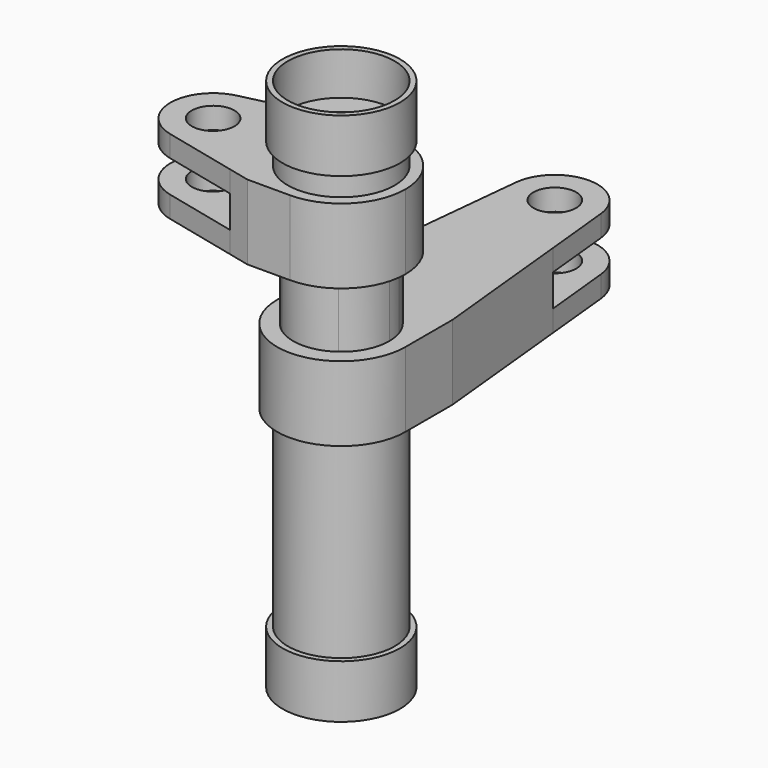
from build123d import *

# Parameters (mm, degrees)
F1_START       = 20
F0_R           = 5.5
F0_R_2         = 5
F1_DEPTH       = 5
F2_START       = 18
F0_R_3         = 2.75
F2_DEPTH       = 3
F3_START       = 14.5
F3_DEPTH       = 3.5
F4_START       = 11
F0_R_4         = 2
F4_DEPTH       = 7
F5_START       = 13
F5_DEPTH       = 3
F6_START       = 11
F6_DEPTH       = 3.5
F7_START       = 5
F7_DEPTH       = 6
F8_START       = 1.5
F8_DEPTH       = 3.5
F9_DEPTH       = 5
F9_DEPTH_BACK  = 2
F10_DEPTH      = 3
F11_DEPTH      = 1.5
F11_DEPTH_BACK = 2
F12_START      = -2
F12_DEPTH      = 19
F13_START      = -20
F13_DEPTH      = 5


# Not quite as in the source:
# - a feature names something its author has since deleted; it is built from what else it names


with BuildPart() as f1:
    # F0 (on Top) → F1 (new body)
    with BuildSketch(Plane.XY.offset(F1_START)):
        Circle(F0_R)
        Circle(F0_R_2, mode=Mode.SUBTRACT)
    extrude(amount=F1_DEPTH)

    # F0 (on Top) → F2 (join)
    with BuildSketch(Plane.XY.offset(F2_START)):
        Circle(F0_R_2)
        with BuildLine():
            ThreePointArc((4.2797543233, 1.3905764747), (4.4445975327, 0.7039550927), (4.5, 0))
            ThreePointArc((4.5, 0), (4.0095293588, -2.0429572488), (2.6450336353, -3.6405764747))
            ThreePointArc((2.6450336353, -3.6405764747), (0, -4.5), (-2.6450336353, -3.6405764747))
            ThreePointArc((-2.6450336353, -3.6405764747), (-4.2797543233, -1.3905764747), (-4.2797543233, 1.3905764747))
            ThreePointArc((-4.2797543233, 1.3905764747), (-2.6450336353, 3.6405764747), (0, 4.5))
            ThreePointArc((0, 4.5), (2.6450336353, 3.6405764747), (4.2797543233, 1.3905764747))
        make_face(mode=Mode.SUBTRACT)
        Polygon((2.6450336353, -3.6405764747), (4.2797543233, 1.3905764747), (0, 4.5), (-4.2797543233, 1.3905764747), (-2.6450336353, -3.6405764747), align=None)
        Circle(F0_R_3, mode=Mode.SUBTRACT)
        with BuildLine():
            Line((-4.2797543233, 1.3905764747), (0, 4.5))
            ThreePointArc((0, 4.5), (-2.6450336353, 3.6405764747), (-4.2797543233, 1.3905764747))
        make_face()
        with BuildLine():
            Line((0, 4.5), (4.2797543233, 1.3905764747))
            ThreePointArc((4.2797543233, 1.3905764747), (2.6450336353, 3.6405764747), (0, 4.5))
        make_face()
        with BuildLine():
            ThreePointArc((2.6450336353, -3.6405764747), (4.0095293588, -2.0429572488), (4.5, 0))
            ThreePointArc((4.5, 0), (4.4445975327, 0.7039550927), (4.2797543233, 1.3905764747))
            Line((4.2797543233, 1.3905764747), (2.6450336353, -3.6405764747))
        make_face()
        with BuildLine():
            ThreePointArc((-4.2797543233, 1.3905764747), (-4.2797543233, -1.3905764747), (-2.6450336353, -3.6405764747))
            Line((-2.6450336353, -3.6405764747), (-4.2797543233, 1.3905764747))
        make_face()
        with BuildLine():
            ThreePointArc((-2.6450336353, -3.6405764747), (0, -4.5), (2.6450336353, -3.6405764747))
            Line((2.6450336353, -3.6405764747), (-2.6450336353, -3.6405764747))
        make_face()
    extrude(amount=F2_DEPTH)

    # F0 (on Top) → F3 (join)
    with BuildSketch(Plane.XY.offset(F3_START)):
        Polygon((2.6450336353, -3.6405764747), (4.2797543233, 1.3905764747), (0, 4.5), (-4.2797543233, 1.3905764747), (-2.6450336353, -3.6405764747), align=None)
        Circle(F0_R_3, mode=Mode.SUBTRACT)
    extrude(amount=F3_DEPTH)


with BuildPart() as f4:
    # F0 (on Top) → F4 (new body)
    with BuildSketch(Plane.XY.offset(F4_START)):
        with BuildLine():
            ThreePointArc((6, 0), (4.2426406871, 4.2426406871), (0, 6))
            ThreePointArc((0, 6), (-4.2426406871, 4.2426406871), (-6, 0))
            ThreePointArc((-6, 0), (-4.2426406871, -4.2426406871), (0, -6))
            ThreePointArc((0, -6), (4.2426406871, -4.2426406871), (6, 0))
        make_face()
        Circle(F0_R, mode=Mode.SUBTRACT)
        Circle(F0_R)
        Circle(F0_R_2, mode=Mode.SUBTRACT)
        with BuildLine():
            Line((-6, -5.5275252317), (-6, 0))
            Line((-6, 0), (-6, 5.5275252317))
            Line((-6, 5.5275252317), (-12.9196363336, 3.8928484448))
            ThreePointArc((-12.9196363336, 3.8928484448), (-16, 0), (-12.9196363336, -3.8928484448))
            Line((-12.9196363336, -3.8928484448), (-6, -5.5275252317))
        make_face()
        with Locations((-12, 0)):
            Circle(F0_R_4, mode=Mode.SUBTRACT)
        Circle(F0_R_2)
        with BuildLine():
            ThreePointArc((4.2797543233, 1.3905764747), (4.4445975327, 0.7039550927), (4.5, 0))
            ThreePointArc((4.5, 0), (4.0095293588, -2.0429572488), (2.6450336353, -3.6405764747))
            ThreePointArc((2.6450336353, -3.6405764747), (0, -4.5), (-2.6450336353, -3.6405764747))
            ThreePointArc((-2.6450336353, -3.6405764747), (-4.2797543233, -1.3905764747), (-4.2797543233, 1.3905764747))
            ThreePointArc((-4.2797543233, 1.3905764747), (-2.6450336353, 3.6405764747), (0, 4.5))
            ThreePointArc((0, 4.5), (2.6450336353, 3.6405764747), (4.2797543233, 1.3905764747))
        make_face(mode=Mode.SUBTRACT)
        with BuildLine():
            ThreePointArc((-6, 0), (-4.2426406871, 4.2426406871), (0, 6))
            Line((0, 6), (-4, 6))
            Line((-4, 6), (-6, 5.5275252317))
            Line((-6, 5.5275252317), (-6, 0))
        make_face()
        with BuildLine():
            ThreePointArc((0, -6), (-4.2426406871, -4.2426406871), (-6, 0))
            Line((-6, 0), (-6, -5.5275252317))
            Line((-6, -5.5275252317), (-4, -6))
            Line((-4, -6), (0, -6))
        make_face()
        with BuildLine():
            ThreePointArc((-4.2797543233, 1.3905764747), (-4.2797543233, -1.3905764747), (-2.6450336353, -3.6405764747))
            Line((-2.6450336353, -3.6405764747), (-4.2797543233, 1.3905764747))
        make_face()
        with BuildLine():
            ThreePointArc((2.6450336353, -3.6405764747), (4.0095293588, -2.0429572488), (4.5, 0))
            ThreePointArc((4.5, 0), (4.4445975327, 0.7039550927), (4.2797543233, 1.3905764747))
            Line((4.2797543233, 1.3905764747), (2.6450336353, -3.6405764747))
        make_face()
        with BuildLine():
            ThreePointArc((-2.6450336353, -3.6405764747), (0, -4.5), (2.6450336353, -3.6405764747))
            Line((2.6450336353, -3.6405764747), (-2.6450336353, -3.6405764747))
        make_face()
        with BuildLine():
            Line((0, 4.5), (4.2797543233, 1.3905764747))
            ThreePointArc((4.2797543233, 1.3905764747), (2.6450336353, 3.6405764747), (0, 4.5))
        make_face()
        with BuildLine():
            Line((-4.2797543233, 1.3905764747), (0, 4.5))
            ThreePointArc((0, 4.5), (-2.6450336353, 3.6405764747), (-4.2797543233, 1.3905764747))
        make_face()
    extrude(amount=F4_DEPTH)

    # F0 (on Top) → F5 (cut)
    with BuildSketch(Plane.XY.offset(F5_START)):
        with BuildLine():
            Line((-6, -5.5275252317), (-6, 0))
            Line((-6, 0), (-6, 5.5275252317))
            Line((-6, 5.5275252317), (-12.9196363336, 3.8928484448))
            ThreePointArc((-12.9196363336, 3.8928484448), (-16, 0), (-12.9196363336, -3.8928484448))
            Line((-12.9196363336, -3.8928484448), (-6, -5.5275252317))
        make_face()
        with Locations((-12, 0)):
            Circle(F0_R_4, mode=Mode.SUBTRACT)
    extrude(amount=F5_DEPTH, mode=Mode.SUBTRACT)


with BuildPart() as f6:
    # F0 (on Top) → F6 (new body)
    with BuildSketch(Plane.XY.offset(F6_START)):
        Polygon((2.6450336353, -3.6405764747), (4.2797543233, 1.3905764747), (0, 4.5), (-4.2797543233, 1.3905764747), (-2.6450336353, -3.6405764747), align=None)
        Circle(F0_R_3, mode=Mode.SUBTRACT)
    extrude(amount=F6_DEPTH)

    # F0 (on Top) → F7 (join)
    with BuildSketch(Plane.XY.offset(F7_START)):
        with BuildLine():
            Line((0, 4.5), (4.2797543233, 1.3905764747))
            ThreePointArc((4.2797543233, 1.3905764747), (2.6450336353, 3.6405764747), (0, 4.5))
        make_face()
        Polygon((2.6450336353, -3.6405764747), (4.2797543233, 1.3905764747), (0, 4.5), (-4.2797543233, 1.3905764747), (-2.6450336353, -3.6405764747), align=None)
        Circle(F0_R_3, mode=Mode.SUBTRACT)
        with BuildLine():
            ThreePointArc((2.6450336353, -3.6405764747), (4.0095293588, -2.0429572488), (4.5, 0))
            ThreePointArc((4.5, 0), (4.4445975327, 0.7039550927), (4.2797543233, 1.3905764747))
            Line((4.2797543233, 1.3905764747), (2.6450336353, -3.6405764747))
        make_face()
        with BuildLine():
            Line((-4.2797543233, 1.3905764747), (0, 4.5))
            ThreePointArc((0, 4.5), (-2.6450336353, 3.6405764747), (-4.2797543233, 1.3905764747))
        make_face()
        with BuildLine():
            ThreePointArc((-2.6450336353, -3.6405764747), (0, -4.5), (2.6450336353, -3.6405764747))
            Line((2.6450336353, -3.6405764747), (-2.6450336353, -3.6405764747))
        make_face()
        with BuildLine():
            ThreePointArc((-4.2797543233, 1.3905764747), (-4.2797543233, -1.3905764747), (-2.6450336353, -3.6405764747))
            Line((-2.6450336353, -3.6405764747), (-4.2797543233, 1.3905764747))
        make_face()
    extrude(amount=F7_DEPTH)

    # F0 (on Top) → F8 (join)
    with BuildSketch(Plane.XY.offset(F8_START)):
        Polygon((2.6450336353, -3.6405764747), (4.2797543233, 1.3905764747), (0, 4.5), (-4.2797543233, 1.3905764747), (-2.6450336353, -3.6405764747), align=None)
        Circle(F0_R_3, mode=Mode.SUBTRACT)
    extrude(amount=F8_DEPTH)


with BuildPart() as f9:
    # F0 (on Top) → F9 (new body, two sides)
    with BuildSketch(Plane.XY) as f9_sk:
        with BuildLine():
            Line((-4, 6), (0, 6))
            ThreePointArc((0, 6), (4.2426406871, 4.2426406871), (6, 0))
            Line((6, 0), (6, 5.5275252317))
            Line((6, 5.5275252317), (4.6305157529, 19))
            Line((4.6305157529, 19), (-4.6305157529, 19))
            Line((-4.6305157529, 19), (-6, 5.5275252317))
            Line((-6, 5.5275252317), (-4, 6))
        make_face()
        with BuildLine():
            ThreePointArc((6, 0), (4.2426406871, 4.2426406871), (0, 6))
            ThreePointArc((0, 6), (-4.2426406871, 4.2426406871), (-6, 0))
            ThreePointArc((-6, 0), (-4.2426406871, -4.2426406871), (0, -6))
            ThreePointArc((0, -6), (4.2426406871, -4.2426406871), (6, 0))
        make_face()
        Circle(F0_R, mode=Mode.SUBTRACT)
        Circle(F0_R)
        Circle(F0_R_2, mode=Mode.SUBTRACT)
        Circle(F0_R_2)
        with BuildLine():
            ThreePointArc((4.2797543233, 1.3905764747), (4.4445975327, 0.7039550927), (4.5, 0))
            ThreePointArc((4.5, 0), (4.0095293588, -2.0429572488), (2.6450336353, -3.6405764747))
            ThreePointArc((2.6450336353, -3.6405764747), (0, -4.5), (-2.6450336353, -3.6405764747))
            ThreePointArc((-2.6450336353, -3.6405764747), (-4.2797543233, -1.3905764747), (-4.2797543233, 1.3905764747))
            ThreePointArc((-4.2797543233, 1.3905764747), (-2.6450336353, 3.6405764747), (0, 4.5))
            ThreePointArc((0, 4.5), (2.6450336353, 3.6405764747), (4.2797543233, 1.3905764747))
        make_face(mode=Mode.SUBTRACT)
        with BuildLine():
            Line((-3.9794931225, 25.4045175988), (-4.6305157529, 19))
            Line((-4.6305157529, 19), (4.6305157529, 19))
            Line((4.6305157529, 19), (3.9794931225, 25.4045175988))
            ThreePointArc((3.9794931225, 25.4045175988), (0, 29), (-3.9794931225, 25.4045175988))
        make_face()
        with Locations((0, 25)):
            Circle(F0_R_4, mode=Mode.SUBTRACT)
        with BuildLine():
            ThreePointArc((-6, 0), (-4.2426406871, 4.2426406871), (0, 6))
            Line((0, 6), (-4, 6))
            Line((-4, 6), (-6, 5.5275252317))
            Line((-6, 5.5275252317), (-6, 0))
        make_face()
        with BuildLine():
            ThreePointArc((2.6450336353, -3.6405764747), (4.0095293588, -2.0429572488), (4.5, 0))
            ThreePointArc((4.5, 0), (4.4445975327, 0.7039550927), (4.2797543233, 1.3905764747))
            Line((4.2797543233, 1.3905764747), (2.6450336353, -3.6405764747))
        make_face()
        with BuildLine():
            ThreePointArc((-4.2797543233, 1.3905764747), (-4.2797543233, -1.3905764747), (-2.6450336353, -3.6405764747))
            Line((-2.6450336353, -3.6405764747), (-4.2797543233, 1.3905764747))
        make_face()
        with BuildLine():
            Line((-4.2797543233, 1.3905764747), (0, 4.5))
            ThreePointArc((0, 4.5), (-2.6450336353, 3.6405764747), (-4.2797543233, 1.3905764747))
        make_face()
        with BuildLine():
            ThreePointArc((-2.6450336353, -3.6405764747), (0, -4.5), (2.6450336353, -3.6405764747))
            Line((2.6450336353, -3.6405764747), (-2.6450336353, -3.6405764747))
        make_face()
        with BuildLine():
            Line((0, 4.5), (4.2797543233, 1.3905764747))
            ThreePointArc((4.2797543233, 1.3905764747), (2.6450336353, 3.6405764747), (0, 4.5))
        make_face()
    extrude(amount=F9_DEPTH)
    extrude(f9_sk.sketch, amount=-F9_DEPTH_BACK)

    # F0 (on Top) → F10 (cut)
    with BuildSketch(Plane.XY):
        with BuildLine():
            Line((-3.9794931225, 25.4045175988), (-4.6305157529, 19))
            Line((-4.6305157529, 19), (4.6305157529, 19))
            Line((4.6305157529, 19), (3.9794931225, 25.4045175988))
            ThreePointArc((3.9794931225, 25.4045175988), (0, 29), (-3.9794931225, 25.4045175988))
        make_face()
        with Locations((0, 25)):
            Circle(F0_R_4, mode=Mode.SUBTRACT)
    extrude(amount=F10_DEPTH, mode=Mode.SUBTRACT)


with BuildPart() as f11:
    # F0 (on Top) → F11 (new body, two sides)
    with BuildSketch(Plane.XY) as f11_sk:
        Polygon((2.6450336353, -3.6405764747), (4.2797543233, 1.3905764747), (0, 4.5), (-4.2797543233, 1.3905764747), (-2.6450336353, -3.6405764747), align=None)
        Circle(F0_R_3, mode=Mode.SUBTRACT)
    extrude(amount=F11_DEPTH)
    extrude(f11_sk.sketch, amount=-F11_DEPTH_BACK)

    # F0 (on Top) → F12 (join)
    with BuildSketch(Plane.XY.offset(F12_START)):
        Circle(F0_R_2)
        with BuildLine():
            ThreePointArc((4.2797543233, 1.3905764747), (4.4445975327, 0.7039550927), (4.5, 0))
            ThreePointArc((4.5, 0), (4.0095293588, -2.0429572488), (2.6450336353, -3.6405764747))
            ThreePointArc((2.6450336353, -3.6405764747), (0, -4.5), (-2.6450336353, -3.6405764747))
            ThreePointArc((-2.6450336353, -3.6405764747), (-4.2797543233, -1.3905764747), (-4.2797543233, 1.3905764747))
            ThreePointArc((-4.2797543233, 1.3905764747), (-2.6450336353, 3.6405764747), (0, 4.5))
            ThreePointArc((0, 4.5), (2.6450336353, 3.6405764747), (4.2797543233, 1.3905764747))
        make_face(mode=Mode.SUBTRACT)
        Polygon((2.6450336353, -3.6405764747), (4.2797543233, 1.3905764747), (0, 4.5), (-4.2797543233, 1.3905764747), (-2.6450336353, -3.6405764747), align=None)
        Circle(F0_R_3, mode=Mode.SUBTRACT)
        with BuildLine():
            ThreePointArc((-2.6450336353, -3.6405764747), (0, -4.5), (2.6450336353, -3.6405764747))
            Line((2.6450336353, -3.6405764747), (-2.6450336353, -3.6405764747))
        make_face()
        with BuildLine():
            Line((-4.2797543233, 1.3905764747), (0, 4.5))
            ThreePointArc((0, 4.5), (-2.6450336353, 3.6405764747), (-4.2797543233, 1.3905764747))
        make_face()
        with BuildLine():
            ThreePointArc((-4.2797543233, 1.3905764747), (-4.2797543233, -1.3905764747), (-2.6450336353, -3.6405764747))
            Line((-2.6450336353, -3.6405764747), (-4.2797543233, 1.3905764747))
        make_face()
        with BuildLine():
            Line((0, 4.5), (4.2797543233, 1.3905764747))
            ThreePointArc((4.2797543233, 1.3905764747), (2.6450336353, 3.6405764747), (0, 4.5))
        make_face()
        with BuildLine():
            ThreePointArc((2.6450336353, -3.6405764747), (4.0095293588, -2.0429572488), (4.5, 0))
            ThreePointArc((4.5, 0), (4.4445975327, 0.7039550927), (4.2797543233, 1.3905764747))
            Line((4.2797543233, 1.3905764747), (2.6450336353, -3.6405764747))
        make_face()
    extrude(amount=-F12_DEPTH)

    # F0 (on Top) → F13 (join)
    with BuildSketch(Plane.XY.offset(F13_START)):
        Circle(F0_R)
        Circle(F0_R_2, mode=Mode.SUBTRACT)
    extrude(amount=-F13_DEPTH)


solid = Compound([f1.part, f4.part, f6.part, f9.part, f11.part])
